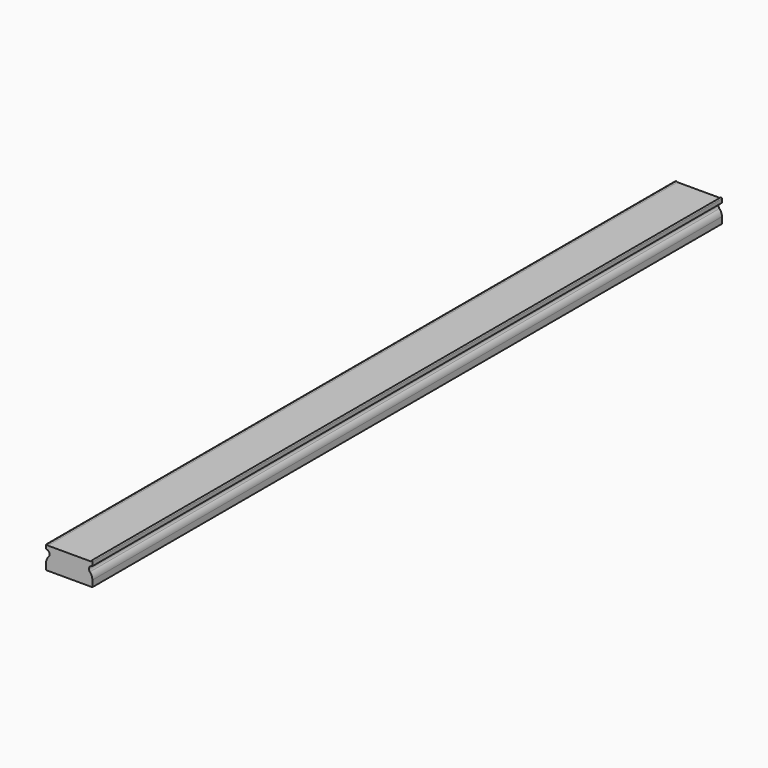
from build123d import *

# Parameters (mm, degrees)
F1_DEPTH = 215.9
F2_R     = 2.54
F3_W     = 12.192
F3_H     = 0.254
F4_DEPTH = 215.901
F5_R     = 0.25399


# Not quite as in the source:
# - a fillet or chamfer is up to 0.001 mm smaller than in the source, because OpenCascade refuses the exact size


with BuildPart() as f1:
    # F0 (on Front) → F1 (new body)
    with BuildSketch(Plane.XZ):
        with BuildLine():
            Line((10.5184665114, -10.1497577667), (4.1684665114, -10.1497577667))
            Line((4.1684665114, -10.1497577667), (4.1684665114, -11.4197577667))
            ThreePointArc((4.1684665114, -11.4197577667), (4.8419857204, -11.6987385576), (5.1209665114, -12.3722577667))
            ThreePointArc((5.1209665114, -12.3722577667), (4.8419857204, -13.0457769758), (4.1684665114, -13.3247577667))
            Line((4.1684665114, -13.3247577667), (4.1684665114, -16.4997577667))
            Line((4.1684665114, -16.4997577667), (10.5184665114, -16.4997577667))
            Line((10.5184665114, -16.4997577667), (10.5184665114, -10.1497577667))
        make_face()
        with BuildLine():
            Line((16.8684665114, -10.1497577667), (10.5184665114, -10.1497577667))
            Line((10.5184665114, -10.1497577667), (10.5184665114, -16.4997577667))
            Line((10.5184665114, -16.4997577667), (16.8684665114, -16.4997577667))
            Line((16.8684665114, -16.4997577667), (16.8684665114, -13.3247577667))
            ThreePointArc((16.8684665114, -13.3247577667), (15.9159665114, -12.3722577667), (16.8684665114, -11.4197577667))
            Line((16.8684665114, -11.4197577667), (16.8684665114, -10.1497577667))
        make_face()
    extrude(amount=F1_DEPTH)

    # F2
    f2_edges = [f1.edges().sort_by_distance(p)[0] for p in [
        (16.868467, -107.95, -13.324758),
        (4.168467, -107.95, -13.324758),
    ]]
    fillet(f2_edges, radius=F2_R)

    # F3 (on face) → F4 (cut, through all)
    with BuildSketch(Plane.XZ.offset(215.9)):
        with Locations((10.5184665114, -10.2767577667)):
            Rectangle(F3_W, F3_H)
    extrude(amount=-F4_DEPTH, mode=Mode.SUBTRACT)

    # F5 (radius 0.254 in the source; OpenCascade refuses exactly that, so slightly less here)
    f5_edges = [f1.edges().sort_by_distance(p)[0] for p in [
        (4.422467, -107.95, -10.403758),
        (16.614467, -107.95, -10.403758),
        (16.868467, -107.95, -10.149758),
        (4.168467, -107.95, -10.149758),
    ]]
    fillet(f5_edges, radius=F5_R)


solid = f1.part
